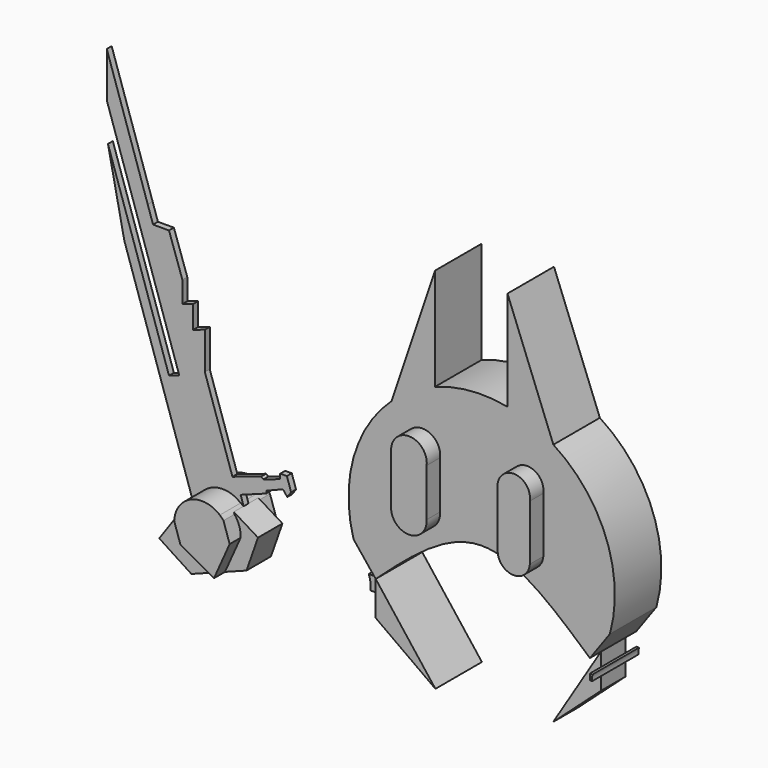
from build123d import *

# Parameters (mm, degrees)
F1_DEPTH = 4.826
F2_DEPTH = 2.54
F3_DEPTH = 4.318
F4_DEPTH = 0.508
F5_DEPTH = 7.62


# Not quite as in the source:
# - a feature names something its author has since deleted; it is built from what else it names


with BuildPart() as f1:
    # F0 (on Front) → F1 (new body, symmetric)
    with BuildSketch(Plane.XZ):
        with BuildLine():
            Line((-19.4491906807, 11.888597546), (-15.762093921, 7.2797275278))
            add(Edge.make_bspline(
                [(-15.762093921, 7.2797275278), (-13.7826219563, 9.0675403506), (-11.8031481855, 10.8553523876), (-9.8214397399, 12.4394689606)],
                knots=[0, 0, 0, 0, 0.1685559759, 0.1685559759, 0.1685559759, 0.1685559759], degree=3))
            add(Edge.make_bspline(
                [(-9.8214397399, 12.4394689606), (-5.9471315119, 15.5364713912), (1.8450447155, 20.1891726215), (9.7388153599, 15.5763916719), (13.7078197829, 12.4716475158)],
                knots=[0.1685559759, 0.1685559759, 0.1685559759, 0.1685559759, 0.4980887111, 0.8298685344, 0.8298685344, 0.8298685344, 0.8298685344], degree=3))
            add(Edge.make_bspline(
                [(13.7078197829, 12.4716475158), (15.7430627116, 10.8795836338), (17.780595361, 9.0796552071), (19.8181439191, 7.2797275278)],
                knots=[0.8298685344, 0.8298685344, 0.8298685344, 0.8298685344, 1, 1, 1, 1], degree=3))
            Line((19.8181439191, 7.2797275278), (23.1367782905, 11.888597546))
            ThreePointArc((23.1367782905, 11.888597546), (22.5103556775, 25.7526809049), (13.747217288, 36.5143080234))
            ThreePointArc((13.747217288, 36.5143080234), (10.0801885199, 38.3998252427), (6.1269021237, 39.571918174))
            ThreePointArc((6.1269021237, 39.571918174), (0.0427353837, 39.9171387541), (-5.9047092104, 38.5889200339))
            ThreePointArc((-5.9047092104, 38.5889200339), (-9.7419423832, 36.7133942622), (-13.1471515298, 34.135312415))
            ThreePointArc((-13.1471515298, 34.135312415), (-19.4367130362, 23.9010396945), (-19.4491906807, 11.888597546))
        make_face()
        with BuildLine():
            ThreePointArc((-5.0697573461, 20.5555651337), (-7.9242470393, 17.4173960024), (-10.9691116959, 20.37120983))
            Line((-10.9691116959, 20.37120983), (-10.9691116959, 28.851531446))
            ThreePointArc((-10.9691116959, 28.851531446), (-7.8231993673, 31.8069640078), (-5.0697573461, 28.482824564))
            Line((-5.0697573461, 28.482824564), (-5.0697573461, 20.5555651337))
        make_face(mode=Mode.SUBTRACT)
        with BuildLine():
            ThreePointArc((6.7289490253, 28.851531446), (9.4020958059, 31.9821073356), (12.0752425864, 28.851531446))
            Line((12.0752425864, 28.851531446), (12.0752425864, 19.6337904781))
            ThreePointArc((12.0752425864, 19.6337904781), (9.3130419135, 17.1434102004), (6.7289490253, 19.8181457818))
            Line((6.7289490253, 19.8181457818), (6.7289490253, 28.851531446))
        make_face(mode=Mode.SUBTRACT)
        with BuildLine():
            Line((6.1269021237, 56.1337606095), (6.1269021237, 39.571918174))
            ThreePointArc((6.1269021237, 39.571918174), (10.0801885199, 38.3998252427), (13.747217288, 36.5143080234))
            Line((13.747217288, 36.5143080234), (6.1269021237, 56.1337606095))
        make_face()
        with BuildLine():
            Line((-5.9047092104, 55.5806973326), (-13.1471515298, 34.135312415))
            ThreePointArc((-13.1471515298, 34.135312415), (-9.7419423832, 36.7133942622), (-5.9047092104, 38.5889200339))
            Line((-5.9047092104, 38.5889200339), (-5.9047092104, 55.5806973326))
        make_face()
    extrude(amount=F1_DEPTH, both=True)

    # F0 (on Front) → F5 (join)
    with BuildSketch(Plane.XZ):
        with BuildLine():
            Line((-10.9691116959, 28.851531446), (-10.9691116959, 20.37120983))
            ThreePointArc((-10.9691116959, 20.37120983), (-7.9242470393, 17.4173960024), (-5.0697573461, 20.5555651337))
            Line((-5.0697573461, 20.5555651337), (-5.0697573461, 28.482824564))
            ThreePointArc((-5.0697573461, 28.482824564), (-7.8231993673, 31.8069640078), (-10.9691116959, 28.851531446))
        make_face()
        with BuildLine():
            Line((12.0752425864, 19.6337904781), (12.0752425864, 28.851531446))
            ThreePointArc((12.0752425864, 28.851531446), (9.4020958059, 31.9821073356), (6.7289490253, 28.851531446))
            Line((6.7289490253, 28.851531446), (6.7289490253, 19.8181457818))
            ThreePointArc((6.7289490253, 19.8181457818), (9.3130419135, 17.1434102004), (12.0752425864, 19.6337904781))
        make_face()
    extrude(amount=F5_DEPTH)


with BuildPart() as f1b:
    # F0 (on Front) → F1, piece 2 (new body, symmetric)
    with BuildSketch(Plane.XZ):
        with BuildLine():
            Line((20.256677791, 5.0279753847), (19.8181439191, 5.0279753847))
            Line((19.8181439191, 5.0279753847), (19.8181439191, 4.0157617505))
            Line((19.8181439191, 4.0157617505), (20.1839942505, 4.0157617505))
            ThreePointArc((20.1839942505, 4.0157617505), (20.1659410394, 4.525774482), (20.256677791, 5.0279753847))
        make_face()
    extrude(amount=F1_DEPTH, both=True)


with BuildPart() as f1c:
    # F0 (on Front) → F1, piece 3 (new body, symmetric)
    with BuildSketch(Plane.XZ):
        Polygon((-5.842322018, -5.5659487844), (-15.762093921, 7.2797275278), (-15.762093921, 4.9683086441), (-15.762093921, 1.5670161229), align=None)
    extrude(amount=F1_DEPTH, both=True)


with BuildPart() as f1d:
    # F0 (on Front) → F1, piece 4 (new body, symmetric)
    with BuildSketch(Plane.XZ):
        with BuildLine():
            Line((-48.2102003072, 1.7716179376), (-42.6312641226, -1.3567452536))
            Line((-42.6312641226, -1.3567452536), (-40.025416848, 4.4845512796))
            Line((-40.025416848, 4.4845512796), (-41.0539040545, 7.5874454587))
            ThreePointArc((-41.0539040545, 7.5874454587), (-41.3406632708, 7.908442582), (-41.6561064599, 8.2013002196))
            ThreePointArc((-41.6561064599, 8.2013002196), (-46.4845280708, 8.9017869639), (-49.2386875136, 4.8745121166))
            Line((-49.2386875136, 4.8745121166), (-48.2102003072, 1.7716179376))
        make_face()
    extrude(amount=F1_DEPTH, both=True)


with BuildPart() as f2:
    # F0 (on Front) → F2 (new body, symmetric)
    with BuildSketch(Plane.XZ):
        Polygon((19.8181439191, 7.2797275278), (11.8864420801, -5.5659487844), (19.8181439191, 1.5670161229), (19.8181439191, 4.0157617505), (19.8181439191, 5.0279753847), align=None)
    extrude(amount=F2_DEPTH, both=True)


with BuildPart() as f2b:
    # F0 (on Front) → F2, piece 2 (new body, symmetric)
    with BuildSketch(Plane.XZ):
        with BuildLine():
            Line((-44.6452607465, -2.1211398475), (-42.6312641226, -1.3567452536))
            Line((-42.6312641226, -1.3567452536), (-48.2102003072, 1.7716179376))
            ThreePointArc((-48.2102003072, 1.7716179376), (-49.0086556744, 3.2288600216), (-49.2386875136, 4.8745121166))
            Line((-49.2386875136, 4.8745121166), (-49.5244317276, 5.7365880401))
            Line((-49.5244317276, 5.7365880401), (-53.5550825298, 0))
            Line((-53.5550825298, 0), (-48.2102003072, -3.4741811065))
            Line((-48.2102003072, -3.4741811065), (-44.6452607465, -2.1211398475))
        make_face()
    extrude(amount=F2_DEPTH, both=True)


with BuildPart() as f2c:
    # F0 (on Front) → F2, piece 3 (new body, symmetric)
    with BuildSketch(Plane.XZ):
        with BuildLine():
            Line((-42.6312641226, -1.3567452536), (-41.2408662619, -0.8290320512))
            Line((-41.2408662619, -0.8290320512), (-39.0565654234, 0))
            Line((-39.0565654234, 0), (-37.1474996209, 5.4384674877))
            Line((-37.1474996209, 5.4384674877), (-41.1557403652, 7.8946804868))
            Line((-41.1557403652, 7.8946804868), (-41.0539040545, 7.5874454587))
            ThreePointArc((-41.0539040545, 7.5874454587), (-40.2554486873, 6.1302033746), (-40.025416848, 4.4845512796))
            Line((-40.025416848, 4.4845512796), (-42.6312641226, -1.3567452536))
        make_face()
    extrude(amount=F2_DEPTH, both=True)


with BuildPart() as f3:
    # F0 (on Front) → F3 (new body, symmetric)
    with BuildSketch(Plane.XZ):
        with BuildLine():
            Line((-15.762093921, 4.9683086441), (-15.762093921, 7.2797275278))
            Line((-15.762093921, 7.2797275278), (-17.3304833915, 7.2797275278))
            ThreePointArc((-17.3304833915, 7.2797275278), (-17.0896080002, 6.4576904492), (-17.0083409329, 5.6049527542))
            ThreePointArc((-17.0083409329, 5.6049527542), (-17.0196339379, 5.2858324269), (-17.0534564546, 4.9683086441))
            Line((-17.0534564546, 4.9683086441), (-15.762093921, 4.9683086441))
        make_face()
    extrude(amount=F3_DEPTH, both=True)


with BuildPart() as f4:
    # F0 (on Front) → F4 (new body, symmetric)
    with BuildSketch(Plane.XZ):
        with BuildLine():
            Line((-41.6561064599, 8.2013002196), (-41.1557403652, 7.8946804868))
            Line((-41.1557403652, 7.8946804868), (-41.6561064599, 9.4042598309))
            Line((-41.6561064599, 9.4042598309), (-37.39515692, 10.978648439))
            Line((-37.39515692, 10.978648439), (-37.39515692, 11.4023303613))
            Line((-37.39515692, 11.4023303613), (-34.6250385046, 12.4941263348))
            Line((-34.6250385046, 12.4941263348), (-33.9080691338, 11.5978755057))
            Line((-33.9080691338, 11.5978755057), (-33.2663303501, 12.5123980251))
            Line((-33.2663303501, 12.5123980251), (-33.9732468128, 14.6451294422))
            Line((-33.9732468128, 14.6451294422), (-35.0756955059, 14.6451294422))
            Line((-35.0756955059, 14.6451294422), (-35.0756955059, 13.8269480115))
            Line((-35.0756955059, 13.8269480115), (-37.8684664491, 12.9012544429))
            Line((-37.8684664491, 12.9012544429), (-38.2543841723, 13.1811112886))
            Line((-38.2543841723, 13.1811112886), (-43.0145218035, 11.6033131517))
            Line((-43.0145218035, 11.6033131517), (-47.5972788614, 25.4292607277))
            Line((-47.5972788614, 25.4292607277), (-47.5972788614, 31.6165960183))
            Line((-47.5972788614, 31.6165960183), (-49.5319052912, 30.9753435561))
            Line((-49.5319052912, 30.9753435561), (-49.5319052912, 34.7506268671))
            Line((-49.5319052912, 34.7506268671), (-51.329412806, 34.1548239244))
            Line((-51.329412806, 34.1548239244), (-51.329412806, 37.700308))
            Line((-51.329412806, 37.700308), (-53.5550825298, 44.1921142478))
            Line((-53.5550825298, 44.1921142478), (-56.2054766065, 44.1921142478))
            Line((-56.2054766065, 44.1921142478), (-57.0860852852, 46.8488663453))
            Line((-57.0860852852, 46.8488663453), (-63.8919092274, 67.3816949129))
            Line((-63.8919092274, 67.3816949129), (-63.8919092274, 59.8809927873))
            Line((-63.8919092274, 59.8809927873), (-51.8436354556, 23.5319567276))
            Line((-51.8436354556, 23.5319567276), (-53.5550825298, 22.9646794314))
            Line((-53.5550825298, 22.9646794314), (-63.6945962906, 53.5550825298))
            Line((-63.6945962906, 53.5550825298), (-60.9696031492, 40.2660946392))
            Line((-60.9696031492, 40.2660946392), (-49.5244317276, 5.7365880401))
            Line((-49.5244317276, 5.7365880401), (-49.2386875136, 4.8745121166))
            ThreePointArc((-49.2386875136, 4.8745121166), (-46.4845280708, 8.9017869639), (-41.6561064599, 8.2013002196))
        make_face()
    extrude(amount=F4_DEPTH, both=True)


solid = Compound([f1.part, f1b.part, f1c.part, f1d.part, f2.part, f2b.part, f2c.part, f3.part, f4.part])
